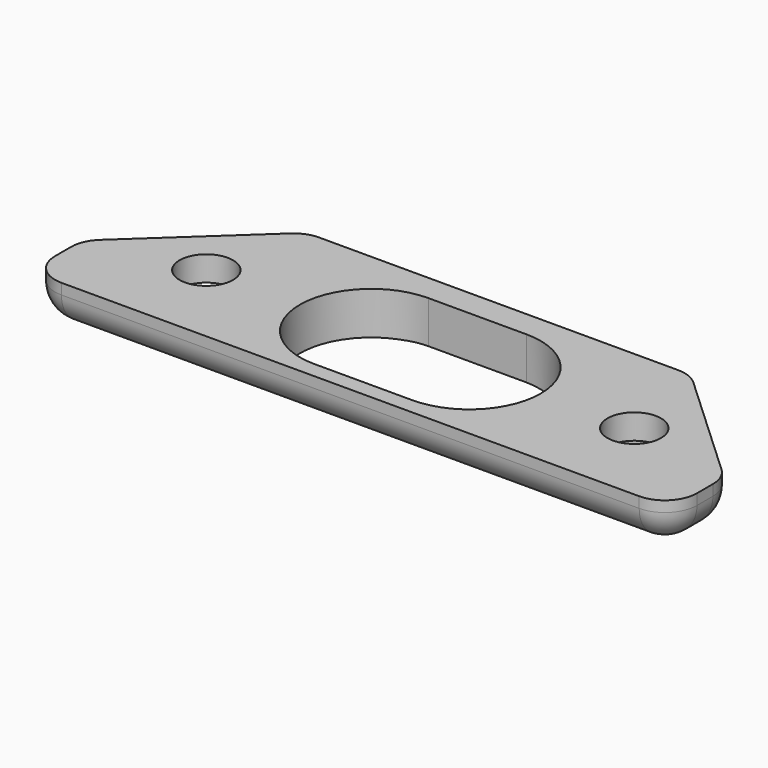
from build123d import *

# Parameters (mm, degrees)
F0_R         = 1.5
F1_DEPTH     = 2.4
F2_DEPTH     = 1
F3_T1_DEPTH  = 1.1190522621
F3_T3_DEPTH  = 32.4
F3_T5_DEPTH  = 20.138628613
F3_T7_DEPTH  = 2.365520331
F3_T9_DEPTH  = 8.3614446785
F3_T11_DEPTH = 8.3614446785
F3_T13_DEPTH = 5.1
F3_T15_DEPTH = 2.5639483811
F3_T20_DEPTH = 1.8
F3_S25_W     = 1.8
F3_S25_H     = 1.8
F3_T26_DEPTH = 1.8
F3_S31_W     = 1.8
F3_S31_H     = 1.8
F3_T32_DEPTH = 1.8
F3_T38_DEPTH = 1.8
F3_T44_DEPTH = 1.8
F3_T50_DEPTH = 1.8


# Not quite as in the source:
# - a fillet or chamfer that OpenCascade refuses, or shapes differently, is made with other operations: its cross-section is extruded or revolved along the edge and cut away or added


with BuildPart() as f1:
    # F0 (on Top) → F1 (new body)
    with BuildSketch(Plane.XY):
        Polygon((-18, -1.2002319389), (-18, -4.9048635534), (18, -4.9048635534), (18, -1.2002319389), (10.7755224389, 5.5), (-10.7755224389, 5.5), align=None)
        Polygon((-9.6294171928, 2.1985610038), (-8.9106989153, -0.9537044309), (-11.2812817225, -3.1522654347), (-14.3705828072, -2.1985610038), (-15.0893010847, 0.9537044309), (-12.7187182775, 3.1522654347), align=None, mode=Mode.SUBTRACT)
        with BuildLine():
            ThreePointArc((-2.75, -4), (-6.75, 0), (-2.75, 4))
            Line((-2.75, 4), (2.75, 4))
            ThreePointArc((2.75, 4), (6.75, 0), (2.75, -4))
            Line((2.75, -4), (-2.75, -4))
        make_face(mode=Mode.SUBTRACT)
        Polygon((9.6294171928, 2.1985610038), (12.7187182775, 3.1522654347), (15.0893010847, 0.9537044309), (14.3705828072, -2.1985610038), (11.2812817225, -3.1522654347), (8.9106989153, -0.9537044309), align=None, mode=Mode.SUBTRACT)
        Polygon((-11.2812817225, -3.1522654347), (-8.9106989153, -0.9537044309), (-9.6294171928, 2.1985610038), (-12.7187182775, 3.1522654347), (-15.0893010847, 0.9537044309), (-14.3705828072, -2.1985610038), align=None)
        with Locations((-12, 0)):
            Circle(F0_R, mode=Mode.SUBTRACT)
        Polygon((15.0893010847, 0.9537044309), (12.7187182775, 3.1522654347), (9.6294171928, 2.1985610038), (8.9106989153, -0.9537044309), (11.2812817225, -3.1522654347), (14.3705828072, -2.1985610038), align=None)
        with Locations((12, 0)):
            Circle(F0_R, mode=Mode.SUBTRACT)
    extrude(amount=F1_DEPTH)

    # F0 (on Top) → F2 (cut)
    with BuildSketch(Plane.XY):
        Polygon((15.0893010847, 0.9537044309), (12.7187182775, 3.1522654347), (9.6294171928, 2.1985610038), (8.9106989153, -0.9537044309), (11.2812817225, -3.1522654347), (14.3705828072, -2.1985610038), align=None)
        with Locations((12, 0)):
            Circle(F0_R, mode=Mode.SUBTRACT)
        Polygon((-11.2812817225, -3.1522654347), (-8.9106989153, -0.9537044309), (-9.6294171928, 2.1985610038), (-12.7187182775, 3.1522654347), (-15.0893010847, 0.9537044309), (-14.3705828072, -2.1985610038), align=None)
        with Locations((-12, 0)):
            Circle(F0_R, mode=Mode.SUBTRACT)
    extrude(amount=F2_DEPTH, mode=Mode.SUBTRACT)

    # F3: fillet of radius 1.8 on 12 edges, made by hand

    # F3_s2 → F3_t1 (cut)
    with BuildSketch(Plane.XZ.offset(1.9858112913)):
        with BuildLine():
            ThreePointArc((-18, 1.8), (-17.4727922061, 0.5272077939), (-16.2, 0))
            Line((-16.2, 0), (-18, 0))
            Line((-18, 0), (-18, 1.8))
        make_face()
        with BuildLine():
            ThreePointArc((16.2, 0), (17.4727922061, 0.5272077939), (18, 1.8))
            Line((18, 1.8), (18, 0))
            Line((18, 0), (16.2, 0))
        make_face()
    extrude(amount=F3_T1_DEPTH, mode=Mode.SUBTRACT)

    # F3_s4 → F3_t3 (cut)
    with BuildSketch(Plane.YZ.offset(-16.2)):
        with BuildLine():
            ThreePointArc((-4.9048635534, 1.8), (-4.3776557595, 0.5272077939), (-3.1048635534, 0))
            Line((-3.1048635534, 0), (-4.9048635534, 0))
            Line((-4.9048635534, 0), (-4.9048635534, 1.8))
        make_face()
    extrude(amount=F3_T3_DEPTH, mode=Mode.SUBTRACT)

    # F3_s6 → F3_t5 (cut)
    with BuildSketch(Plane.YZ.offset(-10.0693143065)):
        with BuildLine():
            ThreePointArc((3.7, 0), (4.9727922061, 0.5272077939), (5.5, 1.8))
            Line((5.5, 1.8), (5.5, 0))
            Line((5.5, 0), (3.7, 0))
        make_face()
    extrude(amount=F3_T5_DEPTH, mode=Mode.SUBTRACT)

    # F3_s8 → F3_t7 (cut)
    with BuildSketch(Plane.XY.offset(1.8)):
        with BuildLine():
            ThreePointArc((10.0693143065, 5.5), (10.7267347006, 5.3756486581), (11.2933205301, 5.0197760282))
            Line((11.2933205301, 5.0197760282), (10.7755224389, 5.5))
            Line((10.7755224389, 5.5), (10.0693143065, 5.5))
        make_face()
        with BuildLine():
            ThreePointArc((-11.2933205301, 5.0197760282), (-10.7267347006, 5.3756486581), (-10.0693143065, 5.5))
            Line((-10.0693143065, 5.5), (-10.7755224389, 5.5))
            Line((-10.7755224389, 5.5), (-11.2933205301, 5.0197760282))
        make_face()
    extrude(amount=F3_T7_DEPTH, mode=Mode.SUBTRACT)

    # F3_s10 → F3_t9 (cut)
    with BuildSketch(Plane(origin=(-3.5684530391, -3.3095075488, 0), x_dir=(0, 0, 1), z_dir=(-0.7332089046, -0.6800034575, 0))):
        with BuildLine():
            ThreePointArc((1.8, 11.3600414903), (0.5272077939, 10.8328336964), (0, 9.5600414903))
            Line((0, 9.5600414903), (0, 11.3600414903))
            Line((0, 11.3600414903), (1.8, 11.3600414903))
        make_face()
    extrude(amount=F3_T9_DEPTH, mode=Mode.SUBTRACT)

    # F3_s12 → F3_t11 (cut)
    with BuildSketch(Plane(origin=(9.6991387326, -8.9953188401, 0), x_dir=(0, 0, 1), z_dir=(-0.7332089046, 0.6800034575, 0))):
        with BuildLine():
            ThreePointArc((0, 9.5600414903), (0.5272077939, 10.8328336964), (1.8, 11.3600414903))
            Line((1.8, 11.3600414903), (0, 11.3600414903))
            Line((0, 11.3600414903), (0, 9.5600414903))
        make_face()
    extrude(amount=F3_T11_DEPTH, mode=Mode.SUBTRACT)

    # F3_s14 → F3_t13 (cut)
    with BuildSketch(Plane.XY.offset(1.8)):
        with BuildLine():
            ThreePointArc((-18, -3.1048635534), (-17.4727922061, -4.3776557595), (-16.2, -4.9048635534))
            Line((-16.2, -4.9048635534), (-18, -4.9048635534))
            Line((-18, -4.9048635534), (-18, -3.1048635534))
        make_face()
        with BuildLine():
            ThreePointArc((16.2, -4.9048635534), (17.4727922061, -4.3776557595), (18, -3.1048635534))
            Line((18, -3.1048635534), (18, -4.9048635534))
            Line((18, -4.9048635534), (16.2, -4.9048635534))
        make_face()
    extrude(amount=F3_T13_DEPTH, mode=Mode.SUBTRACT)

    # F3_s16 → F3_t15 (cut)
    with BuildSketch(Plane.XY.offset(1.8)):
        with BuildLine():
            ThreePointArc((-18, -1.9858112913), (-17.8497289478, -1.265815181), (-17.4240062235, -0.666035263))
            Line((-17.4240062235, -0.666035263), (-18, -1.2002319389))
            Line((-18, -1.2002319389), (-18, -1.9858112913))
        make_face()
        with BuildLine():
            ThreePointArc((18, -1.9858112913), (17.8497289478, -1.265815181), (17.4240062235, -0.666035263))
            Line((17.4240062235, -0.666035263), (18, -1.2002319389))
            Line((18, -1.2002319389), (18, -1.9858112913))
        make_face()
    extrude(amount=F3_T15_DEPTH, mode=Mode.SUBTRACT)


with BuildPart() as f3_tool18:
    # F3_s19 → F3_t20 (new body)
    with BuildSketch(Plane.XY.offset(1.8)):
        Polygon((-16.2, -1.9858112913), (-18, -1.9858112913), (-18, -1.2002319389), (-17.4240062235, -0.666035263), align=None)
    extrude(amount=-F3_T20_DEPTH)

    # F3_s21 → F3_t22 (revolve, cut)
    with BuildSketch(Plane(origin=(-16.2, -1.9858112913, 1.8), x_dir=(0.9165160821, -0.399997839, 0), z_dir=(0.399997839, 0.9165160821, 0))):
        with BuildLine():
            ThreePointArc((0, -1.8), (1.8, 0), (0, 1.8))
            Line((0, 1.8), (0, -1.8))
        make_face()
    revolve(axis=Axis((-16.2, -1.9858112913, 1.8), (0, 0, -1)), mode=Mode.SUBTRACT)


with BuildPart() as f1_1:
    add(f1.part)

    # F3_t17: cut F3_tool18
    add(f3_tool18.part, mode=Mode.SUBTRACT)


with BuildPart() as f3_tool24:
    # F3_s25 → F3_t26 (new body)
    with BuildSketch(Plane.YZ.offset(-16.2)):
        with Locations((-4.0048635534, 0.9)):
            Rectangle(F3_S25_W, F3_S25_H)
    extrude(amount=-F3_T26_DEPTH)

    # F3_s27 → F3_t28 (revolve, cut)
    with BuildSketch(Plane(origin=(-16.2, -3.1048635534, 1.8), x_dir=(0, 0.7071067812, 0.7071067812), z_dir=(0, -0.7071067812, 0.7071067812))):
        with BuildLine():
            ThreePointArc((0, -1.8), (1.8, 0), (0, 1.8))
            Line((0, 1.8), (0, -1.8))
        make_face()
    revolve(axis=Axis((-16.2, -3.1048635534, 1.8), (-1, 0, 0)), mode=Mode.SUBTRACT)


with BuildPart() as f1_2:
    add(f1_1.part)

    # F3_t23: cut F3_tool24
    add(f3_tool24.part, mode=Mode.SUBTRACT)


with BuildPart() as f3_tool30:
    # F3_s31 → F3_t32 (new body)
    with BuildSketch(Plane.XZ.offset(3.1048635534)):
        with Locations((17.1, 0.9)):
            Rectangle(F3_S31_W, F3_S31_H)
    extrude(amount=F3_T32_DEPTH)

    # F3_s33 → F3_t34 (revolve, cut)
    with BuildSketch(Plane(origin=(16.2, -3.1048635534, 1.8), x_dir=(-0.7071067812, 0, 0.7071067812), z_dir=(0.7071067812, 0, 0.7071067812))):
        with BuildLine():
            ThreePointArc((0, -1.8), (1.8, 0), (0, 1.8))
            Line((0, 1.8), (0, -1.8))
        make_face()
    revolve(axis=Axis((16.2, -3.1048635534, 1.8), (0, -1, 0)), mode=Mode.SUBTRACT)


with BuildPart() as f1_3:
    add(f1_2.part)

    # F3_t29: cut F3_tool30
    add(f3_tool30.part, mode=Mode.SUBTRACT)


with BuildPart() as f3_tool36:
    # F3_s37 → F3_t38 (new body)
    with BuildSketch(Plane.XY.offset(1.8)):
        Polygon((16.2, -1.9858112913), (18, -1.9858112913), (18, -1.2002319389), (17.4240062235, -0.666035263), align=None)
    extrude(amount=-F3_T38_DEPTH)

    # F3_s39 → F3_t40 (revolve, cut)
    with BuildSketch(Plane(origin=(16.2, -1.9858112913, 1.8), x_dir=(-0.9165160821, -0.399997839, 0), z_dir=(0.399997839, -0.9165160821, 0))):
        with BuildLine():
            ThreePointArc((0, -1.8), (1.8, 0), (0, 1.8))
            Line((0, 1.8), (0, -1.8))
        make_face()
    revolve(axis=Axis((16.2, -1.9858112913, 1.8), (0, 0, -1)), mode=Mode.SUBTRACT)


with BuildPart() as f1_4:
    add(f1_3.part)

    # F3_t35: cut F3_tool36
    add(f3_tool36.part, mode=Mode.SUBTRACT)


with BuildPart() as f3_tool42:
    # F3_s43 → F3_t44 (new body)
    with BuildSketch(Plane.XY.offset(1.8)):
        Polygon((10.0693143065, 3.7), (10.0693143065, 5.5), (10.7755224389, 5.5), (11.2933205301, 5.0197760282), align=None)
    extrude(amount=-F3_T44_DEPTH)

    # F3_s45 → F3_t46 (revolve, cut)
    with BuildSketch(Plane(origin=(10.0693143065, 3.7, 1.8), x_dir=(-0.3652335523, -0.9309159212, 0), z_dir=(0.9309159212, -0.3652335523, 0))):
        with BuildLine():
            ThreePointArc((0, -1.8), (1.8, 0), (0, 1.8))
            Line((0, 1.8), (0, -1.8))
        make_face()
    revolve(axis=Axis((10.0693143065, 3.7, 1.8), (0, 0, -1)), mode=Mode.SUBTRACT)


with BuildPart() as f1_5:
    add(f1_4.part)

    # F3_t41: cut F3_tool42
    add(f3_tool42.part, mode=Mode.SUBTRACT)


with BuildPart() as f3_tool48:
    # F3_s49 → F3_t50 (new body)
    with BuildSketch(Plane.XY.offset(1.8)):
        Polygon((-10.0693143065, 3.7), (-10.0693143065, 5.5), (-10.7755224389, 5.5), (-11.2933205301, 5.0197760282), align=None)
    extrude(amount=-F3_T50_DEPTH)

    # F3_s51 → F3_t52 (revolve, cut)
    with BuildSketch(Plane(origin=(-10.0693143065, 3.7, 1.8), x_dir=(0.3652335523, -0.9309159212, 0), z_dir=(0.9309159212, 0.3652335523, 0))):
        with BuildLine():
            ThreePointArc((0, -1.8), (1.8, 0), (0, 1.8))
            Line((0, 1.8), (0, -1.8))
        make_face()
    revolve(axis=Axis((-10.0693143065, 3.7, 1.8), (0, 0, -1)), mode=Mode.SUBTRACT)


with BuildPart() as f1_6:
    add(f1_5.part)

    # F3_t47: cut F3_tool48
    add(f3_tool48.part, mode=Mode.SUBTRACT)


solid = f1_6.part
